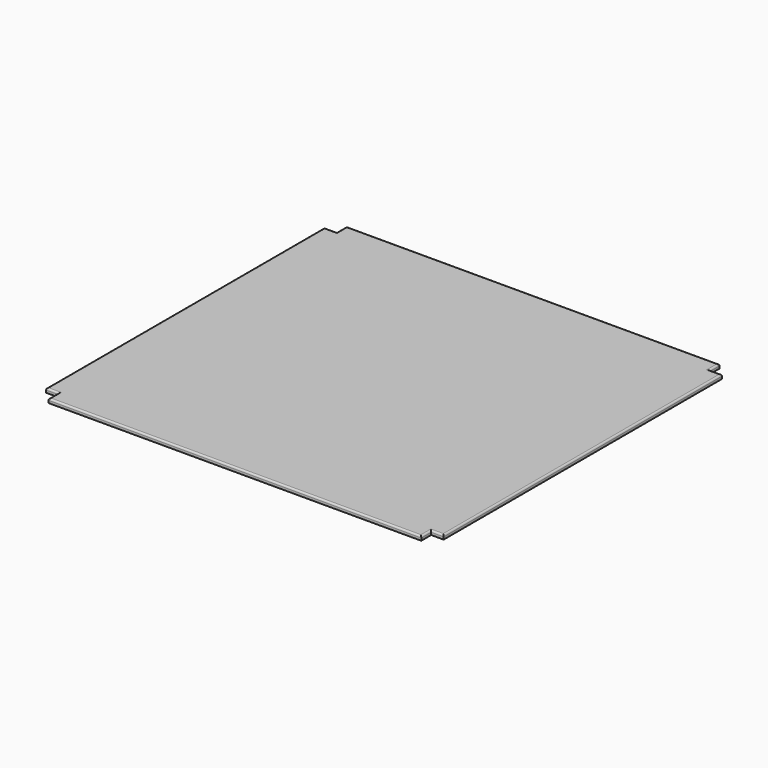
from build123d import *

# Parameters (mm, degrees)
F1_DEPTH = 12.7
F2_R     = 5.08


# Not quite as in the source:
# - a feature names something its author has since deleted; it is built from what else it names


with BuildPart() as f1:
    # F0 (on Top) → F1 (new body)
    with BuildSketch(Plane.XY):
        Polygon((-571.5, -571.5), (571.5, -571.5), (571.5, -533.4), (609.6, -533.4), (609.6, 533.4), (571.5, 533.4), (571.5, 571.5), (-571.5, 571.5), (-571.5, 533.4), (-609.6, 533.4), (-609.6, -533.4), (-571.5, -533.4), align=None)
    extrude(amount=F1_DEPTH)

    # F2
    f2_edges = [f1.edges().sort_by_distance(p)[0] for p in [
        (0, -571.5, 12.7),
        (571.5, -552.45, 12.7),
        (590.55, -533.4, 12.7),
        (609.6, 0, 12.7),
        (590.55, 533.4, 12.7),
        (571.5, 552.45, 12.7),
        (0, 571.5, 12.7),
        (-571.5, 552.45, 12.7),
        (-590.55, 533.4, 12.7),
        (-609.6, 0, 12.7),
        (-590.55, -533.4, 12.7),
        (-571.5, -552.45, 12.7),
    ]]
    fillet(f2_edges, radius=F2_R)


solid = f1.part
